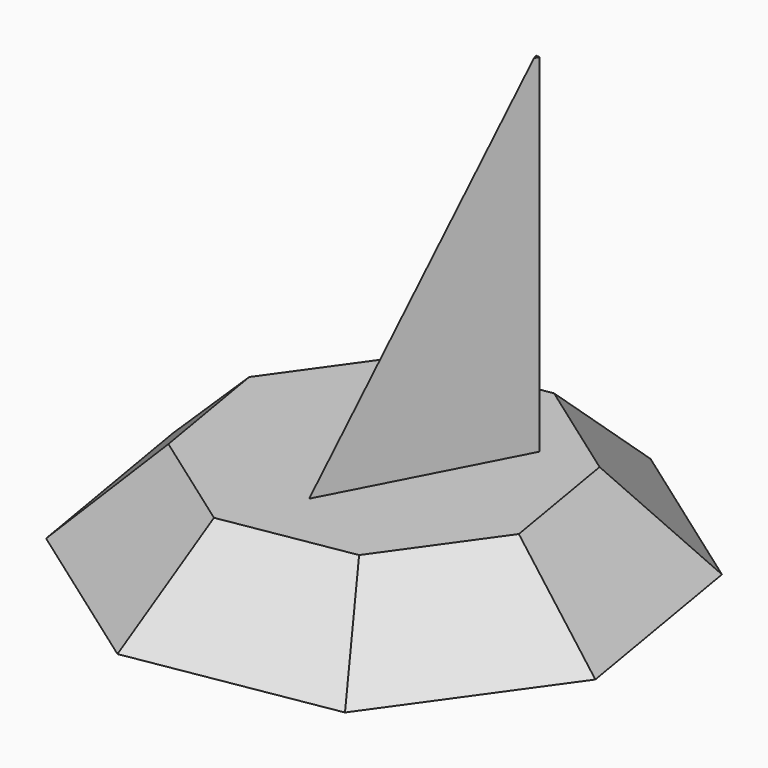
from build123d import *

# Parameters (mm, degrees)
F1_DEPTH = 25.4
F2_SIZE  = 25.39999
F4_DEPTH = 99.314
F5_SIZE2 = 99.2610316746
F5_SIZE  = 40.10406


# Not quite as in the source:
# - a fillet or chamfer is up to 0.001 mm smaller than in the source, because OpenCascade refuses the exact size


with BuildPart() as f1:
    # F0 (on Top) → F1 (new body)
    with BuildSketch(Plane.XY):
        Polygon((40.3215661799, -64.3411021127), (74.0076824868, -16.984376739), (64.3411021127, 40.3215661799), (16.984376739, 74.0076824868), (-40.3215661799, 64.3411021127), (-74.0076824868, 16.984376739), (-64.3411021127, -40.3215661799), (-16.984376739, -74.0076824868), align=None)
    extrude(amount=F1_DEPTH)

    # F2 (size 25.4 in the source; OpenCascade refuses exactly that, so slightly less here)
    f2_edges = [f1.edges().sort_by_distance(p)[0] for p in [
        (11.668595, -69.174392, 25.4),
        (57.164624, -40.662739, 25.4),
        (69.174392, 11.668595, 25.4),
        (40.662739, 57.164624, 25.4),
        (-11.668595, 69.174392, 25.4),
        (-69.174392, -11.668595, 25.4),
        (-40.662739, -57.164624, 25.4),
        (-57.164624, 40.662739, 25.4),
    ]]
    chamfer(f2_edges, length=F2_SIZE)

    # F3 (on face) → F4 (join)
    with BuildSketch(Plane.XY.offset(25.4)):
        Polygon((-18.6424832791, 25.9398680102), (0, -26.7094988376), (25.9398680102, 23.150825873), align=None)
    extrude(amount=F4_DEPTH)

    # F5
    f5_edges = [f1.edges().sort_by_distance(p)[0] for p in [
        (-9.321242, -0.384815, 124.714),
    ]]
    f5_side = f1.faces().sort_by_distance((2.432462, 7.460398, 124.714))[0]
    chamfer(f5_edges, length=F5_SIZE, length2=F5_SIZE2, reference=f5_side)


solid = f1.part
